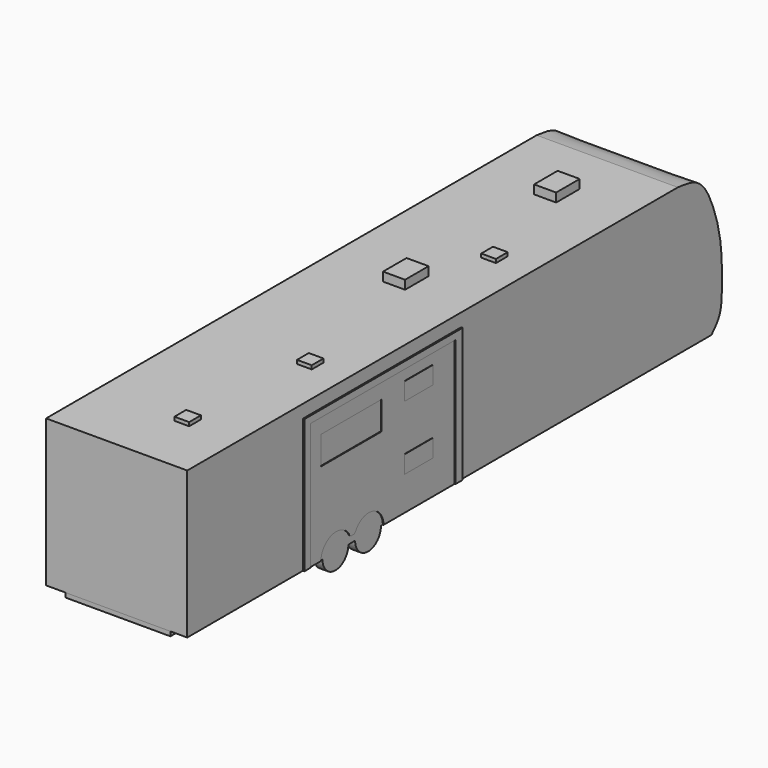
from build123d import *

# Parameters (mm, degrees)
F0_W          = 11582.4
F0_H          = 2540
F1_DEPTH      = 2438.4
F3_DEPTH      = 2438.401
F4_W          = 1738.7323379517
F4_H          = 1235.3963851929
F4_W_2        = 1517.0154571533
F4_H_2        = 1050.2412319183
F5_DEPTH      = 25.4
F4_W_3        = 98.7977981567
F4_H_3        = 270.7209965363
F4_W_4        = 115.3562068939
F4_W_5        = 121.3853359222
F4_W_6        = 111.6482615471
F6_DEPTH      = 25.4
F4_W_7        = 1592.5345420837
F4_H_4        = 643.6148881912
F4_W_8        = 1699.8038291931
F4_W_9        = 1669.4720983505
F4_H_5        = 1913.9534341023
F4_W_10       = 1458.6684703827
F4_H_6        = 455.104470253
F4_W_11       = 1482.0072054863
F4_H_7        = 385.0883245468
F7_DEPTH      = 12.7
F8_R          = 5.08
F9_DEPTH      = 152.4
F11_DEPTH     = 25.4
F10_W         = 1309.9219799042
F10_H         = 488.621711731
F12_DEPTH     = 12.7
F13_DEPTH     = 152.4
F16_W         = 609.6
F16_H         = 304.8
F17_DEPTH     = 6.35
F18_W         = 381
F18_H         = 508
F19_DEPTH     = 152.4
F20_W         = 381
F20_H         = 508
F21_DEPTH     = 152.4
F22_W         = 254
F22_H         = 254
F23_DEPTH     = 63.5
F24_DEPTH     = 76.2
F25_W         = 1815.4902458191
F25_H         = 11320.1663866639
F26_DEPTH     = 76.2
F27_W         = 1015.8215761185
F27_H         = 287.8160476685
F28_DEPTH     = 812.8
F29_R         = 48.2426226407
F29_W         = 291.1487817764
F29_H         = 228.4393310547
F30_DEPTH     = 2692.401
F31_DEPTH     = 1016
F32_DEPTH     = 203.2
F33_W         = 109.7394227982
F33_H         = 105.7481765747
F34_DEPTH     = 101.6
F35_R         = 5.08
F36_T1_DEPTH  = 807.72
F36_T3_DEPTH  = 277.6560476685
F36_T5_DEPTH  = 1005.6615761185
F36_T7_DEPTH  = 280.9887817764
F36_T9_DEPTH  = 218.2793310547
F36_T11_DEPTH = 198.12
F36_S15_W     = 5.1816
F36_S15_H     = 5.1816
F36_T16_DEPTH = 5.1816
F36_S21_W     = 5.1816
F36_S21_H     = 5.1816
F36_T22_DEPTH = 5.1816
F36_S27_W     = 5.1816
F36_S27_H     = 5.1816
F36_T28_DEPTH = 5.1816
F36_S33_W     = 5.1816
F36_S33_H     = 5.1816
F36_T34_DEPTH = 5.1816
F36_S39_W     = 5.1816
F36_S39_H     = 5.1816
F36_T40_DEPTH = 5.1816
F36_S45_W     = 5.1816
F36_S45_H     = 5.1816
F36_T46_DEPTH = 5.1816
F36_S51_W     = 5.1816
F36_S51_H     = 5.1816
F36_T52_DEPTH = 5.1816
F36_S57_W     = 5.1816
F36_S57_H     = 5.1816
F36_T58_DEPTH = 5.1816


# Not quite as in the source:
# - a fillet or chamfer that OpenCascade refuses, or shapes differently, is made with other operations: its cross-section is extruded or revolved along the edge and cut away or added


with BuildPart() as f1:
    # F0 (on Right) → F1 (new body)
    with BuildSketch(Plane.YZ):
        with Locations((5698.256055963, 1234.2060510814)):
            Rectangle(F0_W, F0_H)
    extrude(amount=F1_DEPTH)

    # F2 (on face) → F3 (cut, through all)
    with BuildSketch(Plane.YZ.offset(2438.4)):
        with BuildLine():
            add(Edge.make_bspline(
                [(11227.222442627, -35.7939489186), (11294.0039001697, 34.5419059531), (11441.1259256499, 189.4944004532), (11456.5368861302, 627.4797591897), (11449.8051343447, 1303.5662571069), (11282.6522390087, 1895.0626876843), (11004.4375304796, 2451.3086370719), (10662.2814417447, 2487.1113814171), (10498.9128112793, 2504.2060510814)],
                knots=[0, 0, 0, 0, 0.1266930612, 0.2791095084, 0.4735188477, 0.6617102021, 0.8384774002, 1, 1, 1, 1], degree=3))
            Line((11227.222442627, -35.7939489186), (11489.456055963, -35.7939489186))
            Line((11489.456055963, -35.7939489186), (11489.456055963, 2504.2060510814))
            Line((11489.456055963, 2504.2060510814), (10498.9128112793, 2504.2060510814))
        make_face()
    extrude(amount=-F3_DEPTH, mode=Mode.SUBTRACT)

    # F4 (on face) → F5 (join)
    with BuildSketch(Plane(origin=(0, 0, 0), x_dir=(0, -1, 0), z_dir=(-1, 0, 0))):
        with Locations((-9058.8221549988, 1646.3215351105)):
            Rectangle(F4_W, F4_H)
        with Locations((-9064.6572113037, 1647.0986604691)):
            Rectangle(F4_W_2, F4_H_2, mode=Mode.SUBTRACT)
        Polygon((-6864.5935058594, 234.9270476177), (-6765.7957077026, 234.9270476177), (-6765.7957077026, 2148.88048172), (-5554.6798706055, 2148.88048172), (-2582.3545455933, 2148.88048172), (-2582.3545455933, 234.9270476177), (-2466.9983386993, 234.9270476177), (-2466.9983386993, 2264.0197277069), (-6864.5935058594, 2264.0197277069), align=None)
        Polygon((-2196.6965198517, 2264.0197277069), (-2196.6965198517, 234.9270476177), (-2075.3111839294, 234.9270476177), (-2075.3111839294, 2148.88048172), (-405.8390855789, 2148.88048172), (-405.8390855789, 234.9270476177), (-294.1908240318, 234.9270476177), (-294.1908240318, 2264.0197277069), align=None)
    extrude(amount=F5_DEPTH)

    # F4 (on face) + F5_face (on face) → F6 (join)
    with BuildSketch(Plane(origin=(0, 0, 0), x_dir=(0, -1, 0), z_dir=(-1, 0, 0))):
        with Locations((-6815.194606781, 99.5665493496)):
            Rectangle(F4_W_3, F4_H_3)
        with Locations((-2524.6764421463, 99.5665493496)):
            Rectangle(F4_W_4, F4_H_3)
        with Locations((-2136.0038518906, 99.5665493496)):
            Rectangle(F4_W_5, F4_H_3)
        with Locations((-350.0149548054, 99.5665493496)):
            Rectangle(F4_W_6, F4_H_3)
    with BuildSketch(Plane(origin=(-25.4, 4593.443098287, 1752.5802822759), x_dir=(0, -1, 0), z_dir=(-1, 0, 0))):
        Polygon((-2271.1504075724, -1517.6532346582), (-2172.3526094156, -1517.6532346582), (-2172.3526094156, 396.3001994441), (2011.0885526937, 396.3001994441), (2011.0885526937, -1517.6532346582), (2126.4447595877, -1517.6532346582), (2126.4447595877, 511.439445431), (-2271.1504075724, 511.439445431), align=None)
        Polygon((2396.7465784353, 511.439445431), (2396.7465784353, -1517.6532346582), (2518.1319143576, -1517.6532346582), (2518.1319143576, 396.3001994441), (4187.6040127081, 396.3001994441), (4187.6040127081, -1517.6532346582), (4299.2522742552, -1517.6532346582), (4299.2522742552, 511.439445431), align=None)
    extrude(amount=F6_DEPTH)

    # F4 (on face) → F7 (join)
    with BuildSketch(Plane(origin=(0, 0, 0), x_dir=(0, -1, 0), z_dir=(-1, 0, 0))):
        with BuildLine():
            Line((-6765.7957077026, 2148.88048172), (-6765.7957077026, 234.9270476177))
            Line((-6765.7957077026, 234.9270476177), (-3972.2290414832, 234.9270476177))
            ThreePointArc((-3972.2290414832, 234.9270476177), (-3810.8091471396, 279.2122748766), (-3649.3892527959, 234.9270476177))
            Line((-3649.3892527959, 234.9270476177), (-3268.7322256311, 234.9270476177))
            ThreePointArc((-3268.7322256311, 234.9270476177), (-3106.7426501641, 278.4144938222), (-2944.7530746971, 234.9270476177))
            Line((-2944.7530746971, 234.9270476177), (-2582.3545455933, 234.9270476177))
            Line((-2582.3545455933, 234.9270476177), (-2582.3545455933, 2148.88048172))
            Line((-2582.3545455933, 2148.88048172), (-5554.6798706055, 2148.88048172))
            Line((-5554.6798706055, 2148.88048172), (-6765.7957077026, 2148.88048172))
        make_face()
        with Locations((-5719.4011211395, 1632.1941018105)):
            Rectangle(F4_W_7, F4_H_4, mode=Mode.SUBTRACT)
        with Locations((-3710.1671695709, 1632.1941018105)):
            Rectangle(F4_W_8, F4_H_4, mode=Mode.SUBTRACT)
        with BuildLine():
            Line((-3972.2290414832, 234.9270476177), (-6765.7957077026, 234.9270476177))
            Line((-6765.7957077026, 234.9270476177), (-6765.7957077026, -35.7939489186))
            Line((-6765.7957077026, -35.7939489186), (-4127.1371841431, -35.7939489186))
            ThreePointArc((-4127.1371841431, -35.7939489186), (-4085.3692242957, 119.9863517264), (-3972.2290414832, 234.9270476177))
        make_face()
        with BuildLine():
            Line((-2582.3545455933, 234.9270476177), (-2944.7530746971, 234.9270476177))
            ThreePointArc((-2944.7530746971, 234.9270476177), (-2828.889020926, 120.5433614824), (-2783.4274768829, -35.7939489186))
            Line((-2783.4274768829, -35.7939489186), (-2582.3545455933, -35.7939489186))
            Line((-2582.3545455933, -35.7939489186), (-2582.3545455933, 234.9270476177))
        make_face()
        with Locations((-1240.5751347542, 99.5665493496)):
            Rectangle(F4_W_9, F4_H_3)
        with Locations((-1240.5751347542, 1191.9037646688)):
            Rectangle(F4_W_9, F4_H_5)
        with Locations((-1246.5664148331, 1260.11043787)):
            Rectangle(F4_W_10, F4_H_6, mode=Mode.SUBTRACT)
        with Locations((-1246.5664446354, 1855.2470803261)):
            Rectangle(F4_W_11, F4_H_7, mode=Mode.SUBTRACT)
        with Locations((-9064.6572113037, 1647.0986604691)):
            Rectangle(F4_W_2, F4_H_2)
    extrude(amount=F7_DEPTH)

    # F8
    f8_edges = [f1.edges().sort_by_distance(p)[0] for p in [
        (-12.7, 1987.570047, 1855.24708),
        (-12.7, 1246.566445, 2047.791243),
    ]]
    fillet(f8_edges, radius=F8_R)

    # F4 (on face) → F9 (join)
    with BuildSketch(Plane(origin=(0, 0, 0), x_dir=(0, -1, 0), z_dir=(-1, 0, 0))):
        with BuildLine():
            ThreePointArc((-3528.5879283905, -35.7939489186), (-3807.9879283905, 243.6060510814), (-4087.3879283905, -35.7939489186))
            Line((-4087.3879283905, -35.7939489186), (-3528.5879283905, -35.7939489186))
        make_face()
        with BuildLine():
            Line((-3528.5879283905, -35.7939489186), (-4087.3879283905, -35.7939489186))
            ThreePointArc((-4087.3879283905, -35.7939489186), (-3807.9879283905, -315.1939489186), (-3528.5879283905, -35.7939489186))
        make_face()
        with BuildLine():
            Line((-2828.4271865845, -35.7939489186), (-3387.2271865845, -35.7939489186))
            ThreePointArc((-3387.2271865845, -35.7939489186), (-3107.8271865845, -315.1939489186), (-2828.4271865845, -35.7939489186))
        make_face()
        with BuildLine():
            ThreePointArc((-2828.4271865845, -35.7939489186), (-3107.8271865845, 243.6060510814), (-3387.2271865845, -35.7939489186))
            Line((-3387.2271865845, -35.7939489186), (-2828.4271865845, -35.7939489186))
        make_face()
    extrude(amount=-F9_DEPTH)

    # F10 (on face) → F11 (join)
    with BuildSketch(Plane.YZ.offset(2438.4)):
        Polygon((5663.0005836487, 83.0691084266), (5663.4521484375, -35.7939489186), (5820.454120636, -35.7939489186), (5820.454120636, 231.9672825278), (5663.0005836487, 231.9672825278), align=None)
        Polygon((2402.78840065, -35.7939489186), (2534.1942310333, -35.7939489186), (2541.718006134, 83.0691084266), (2541.718006134, 231.9672825278), (2402.78840065, 231.9672825278), align=None)
        Polygon((2402.78840065, 231.9672825278), (2541.718006134, 231.9672825278), (2541.718006134, 2157.7496528625), (5663.0005836487, 2157.7496528625), (5663.0005836487, 231.9672825278), (5820.454120636, 231.9672825278), (5820.454120636, 2278.1553268433), (2402.78840065, 2278.1553268433), align=None)
    extrude(amount=F11_DEPTH)

    # F10 (on face) → F12 (join)
    with BuildSketch(Plane.YZ.offset(2438.4)):
        with BuildLine():
            Line((2541.718006134, 231.9672825278), (2935.8405070918, 231.9672825278))
            ThreePointArc((2935.8405070918, 231.9672825278), (3105.7881003582, 278.912424909), (3275.7356936245, 231.9672825278))
            Line((3275.7356936245, 231.9672825278), (3637.7238895078, 231.9672825278))
            ThreePointArc((3637.7238895078, 231.9672825278), (3807.7616169979, 280.4213909384), (3977.799344488, 231.9672825278))
            Line((3977.7993444881, 231.9672825278), (5663.0005836487, 231.9672825278))
            Line((5663.0005836487, 231.9672825278), (5663.0005836487, 2157.7496528625))
            Line((5663.0005836487, 2157.7496528625), (2541.718006134, 2157.7496528625))
            Line((2541.718006134, 2157.7496528625), (2541.718006134, 231.9672825278))
        make_face()
        with Locations((3433.8718652725, 1646.3187932968)):
            Rectangle(F10_W, F10_H, mode=Mode.SUBTRACT)
        with BuildLine():
            Line((2534.1942310333, -35.7939489186), (2775.1047611237, -35.7939489186))
            ThreePointArc((2775.1047611237, -35.7939489186), (2821.9186727852, 118.2289442144), (2935.8405070918, 231.9672825278))
            Line((2935.8405070918, 231.9672825278), (2541.718006134, 231.9672825278))
            Line((2541.718006134, 231.9672825278), (2541.718006134, 83.0691084266))
            Line((2541.718006134, 83.0691084266), (2534.1942310333, -35.7939489186))
        make_face()
        with BuildLine():
            Line((3637.7238895078, 231.9672825278), (3275.7356936245, 231.9672825278))
            ThreePointArc((3275.7356936245, 231.9672825278), (3332.4353980139, 189.1756777604), (3378.7021636963, 135.274246335))
            ThreePointArc((3378.7021636963, 135.274246335), (3398.1239015568, 103.4115989251), (3429.4067288236, 83.0691084266))
            Line((3429.4067288236, 83.0691084266), (3487.6588915988, 83.0691084266))
            ThreePointArc((3487.6588915988, 83.0691084266), (3518.9417188656, 103.4115989251), (3538.3634567261, 135.274246335))
            ThreePointArc((3538.3634567261, 135.274246335), (3582.7874836507, 189.021952363), (3637.7238895078, 231.9672825278))
        make_face()
        with BuildLine():
            ThreePointArc((3977.799344488, 231.9672825278), (4088.076710876, 117.4697924054), (4130.2785873413, -35.7939489186))
            Line((4130.2785873413, -35.7939489186), (5663.4521484375, -35.7939489186))
            Line((5663.4521484375, -35.7939489186), (5663.0005836487, 83.0691084266))
            Line((5663.0005836487, 83.0691084266), (5663.0005836487, 231.9672825278))
            Line((5663.0005836487, 231.9672825278), (3977.7993444881, 231.9672825278))
        make_face()
    extrude(amount=F12_DEPTH)

    # F10 (on face) → F13 (join)
    with BuildSketch(Plane.YZ.offset(2438.4)):
        with BuildLine():
            ThreePointArc((2826.7098575592, -35.7939489186), (3106.1098575592, -315.1939489186), (3385.5098575592, -35.7939489186))
            Line((3385.5098575592, -35.7939489186), (2826.7098575592, -35.7939489186))
        make_face()
        with BuildLine():
            Line((2826.7098575592, -35.7939489186), (3385.5098575592, -35.7939489186))
            ThreePointArc((3385.5098575592, -35.7939489186), (3106.1098575592, 243.6060510814), (2826.7098575592, -35.7939489186))
        make_face()
        with BuildLine():
            ThreePointArc((4090.3557628632, -35.7939489186), (3810.9557628632, 243.6060510814), (3531.5557628632, -35.7939489186))
            Line((3531.5557628632, -35.7939489186), (4090.3557628632, -35.7939489186))
        make_face()
        with BuildLine():
            Line((4090.3557628632, -35.7939489186), (3531.5557628632, -35.7939489186))
            ThreePointArc((3531.5557628632, -35.7939489186), (3810.9557628632, -315.1939489186), (4090.3557628632, -35.7939489186))
        make_face()
    extrude(amount=-F13_DEPTH)

    # F16 (on face) → F17 (join)
    with BuildSketch(Plane.YZ.offset(2451.1)):
        with Locations((4881.9495035825, 1817.1032423055)):
            Rectangle(F16_W, F16_H)
        with Locations((4881.9495035825, 706.4627090574)):
            Rectangle(F16_W, F16_H)
    extrude(amount=F17_DEPTH)

    # F18 (on face) → F19 (join)
    with BuildSketch(Plane.XY.offset(2504.2060510814)):
        with Locations((1243.6975836754, 9382.0020343422)):
            Rectangle(F18_W, F18_H)
    extrude(amount=F19_DEPTH)

    # F20 (on face) → F21 (join)
    with BuildSketch(Plane.XY.offset(2504.2060510814)):
        with Locations((1243.6975836754, 6119.3277945057)):
            Rectangle(F20_W, F20_H)
    extrude(amount=F21_DEPTH)

    # F22 (on face) → F23 (join)
    with BuildSketch(Plane.XY.offset(2504.2060510814)):
        with Locations((1778.1576690674, 7366.1090393066)):
            Rectangle(F22_W, F22_H)
        with Locations((1778.1576690674, 3388.5683078766)):
            Rectangle(F22_W, F22_H)
        with Locations((1524.1576690674, 1059.3781728745)):
            Rectangle(F22_W, F22_H)
    extrude(amount=F23_DEPTH)

    # F29 (on face) → F30 (cut, through all)
    with BuildSketch(Plane(origin=(0, 0, -35.7939489186), x_dir=(1, 0, 0), z_dir=(0, 0, -1))):
        with Locations((1222.6868448267, -12362.519959551)):
            Circle(F29_R)
        with Locations((1216.6296839714, -12109.4274520874)):
            Rectangle(F29_W, F29_H)
    extrude(amount=-F30_DEPTH, mode=Mode.SUBTRACT)


with BuildPart() as f24:
    # F14 (on face) → F24 (new body)
    with BuildSketch(Plane(origin=(0, 0, -35.7939489186), x_dir=(1, 0, 0), z_dir=(0, 0, -1))):
        Polygon((1219.2, -11227.222442627), (304.5125207247, -11227.222442627), (1230.4298877716, -12745.1028823853), (2156.3472548186, -11227.222442627), align=None)
    extrude(amount=F24_DEPTH)

    # F27 (on face) → F28 (join)
    with BuildSketch(Plane(origin=(0, 0, -35.7939489186), x_dir=(1, 0, 0), z_dir=(0, 0, -1))):
        with Locations((1225.6785035133, -11765.1133537292)):
            Rectangle(F27_W, F27_H)
    extrude(amount=-F28_DEPTH)

    # F29 (on face) → F31 (join)
    with BuildSketch(Plane(origin=(0, 0, -35.7939489186), x_dir=(1, 0, 0), z_dir=(0, 0, -1))):
        with BuildLine():
            ThreePointArc((1230.3896392389, -12314.8962511959), (1185.9516189301, -12393.7909335936), (1270.9294674674, -12362.519959551))
            ThreePointArc((1270.9294674674, -12362.519959551), (1259.4220707233, -12331.2489855084), (1230.3896392389, -12314.8962511959))
        make_face()
    extrude(amount=-F31_DEPTH)

    # F29 (on face) → F32 (join)
    with BuildSketch(Plane(origin=(0, 0, -35.7939489186), x_dir=(1, 0, 0), z_dir=(0, 0, -1))):
        with Locations((1222.6868448267, -12362.519959551)):
            Circle(F29_R)
        with Locations((1216.6296839714, -12109.4274520874)):
            Rectangle(F29_W, F29_H)
    extrude(amount=-F32_DEPTH)

    # F33 (on face) → F34 (join)
    with BuildSketch(Plane.XY.offset(980.2060510814)):
        with Locations((1221.1564183235, 12363.9168739319)):
            Rectangle(F33_W, F33_H)
    extrude(amount=F34_DEPTH)

    # F35
    f35_edges = [f24.edges().sort_by_distance(p)[0] for p in [
        (1276.02613, 12416.790962, 1031.006051),
        (1276.02613, 12311.042786, 1031.006051),
        (1276.02613, 12363.916874, 1081.806051),
        (1221.156418, 12416.790962, 1081.806051),
        (1166.286707, 12363.916874, 1081.806051),
        (1221.156418, 12311.042786, 1081.806051),
        (1166.286707, 12311.042786, 1031.006051),
        (1166.286707, 12416.790962, 1031.006051),
    ]]
    fillet(f35_edges, radius=F35_R)

    # F36: fillet of radius 5.08 on 16 edges, made by hand

    # F36_s2 → F36_t1 (cut)
    with BuildSketch(Plane.XY.offset(-35.7939489186)):
        with BuildLine():
            ThreePointArc((717.7677154541, 11903.9413775635), (719.2556130057, 11907.5334800119), (722.8477154541, 11909.0213775635))
            Line((722.8477154541, 11909.0213775635), (717.7677154541, 11909.0213775635))
            Line((717.7677154541, 11909.0213775635), (717.7677154541, 11903.9413775635))
        make_face()
        with BuildLine():
            ThreePointArc((717.7677154541, 11626.285329895), (719.2556130057, 11622.6932274466), (722.8477154541, 11621.205329895))
            Line((722.8477154541, 11621.205329895), (717.7677154541, 11621.205329895))
            Line((717.7677154541, 11621.205329895), (717.7677154541, 11626.285329895))
        make_face()
        with BuildLine():
            ThreePointArc((1728.5092915726, 11909.0213775635), (1732.101394021, 11907.5334800119), (1733.5892915726, 11903.9413775635))
            Line((1733.5892915726, 11903.9413775635), (1733.5892915726, 11909.0213775635))
            Line((1733.5892915726, 11909.0213775635), (1728.5092915726, 11909.0213775635))
        make_face()
        with BuildLine():
            ThreePointArc((1728.5092915726, 11621.205329895), (1732.101394021, 11622.6932274466), (1733.5892915726, 11626.285329895))
            Line((1733.5892915726, 11626.285329895), (1733.5892915726, 11621.205329895))
            Line((1733.5892915726, 11621.205329895), (1728.5092915726, 11621.205329895))
        make_face()
    extrude(amount=F36_T1_DEPTH, mode=Mode.SUBTRACT)

    # F36_s4 → F36_t3 (cut)
    with BuildSketch(Plane.XZ.offset(-11903.9413775635)):
        with BuildLine():
            ThreePointArc((717.7677154541, 771.9260510814), (719.2556130057, 775.5181535298), (722.8477154541, 777.0060510814))
            Line((722.8477154541, 777.0060510814), (717.7677154541, 777.0060510814))
            Line((717.7677154541, 777.0060510814), (717.7677154541, 771.9260510814))
        make_face()
        with BuildLine():
            ThreePointArc((1733.5892915726, 771.9260510814), (1732.101394021, 775.5181535298), (1728.5092915726, 777.0060510814))
            Line((1728.5092915726, 777.0060510814), (1733.5892915726, 777.0060510814))
            Line((1733.5892915726, 777.0060510814), (1733.5892915726, 771.9260510814))
        make_face()
    extrude(amount=F36_T3_DEPTH, mode=Mode.SUBTRACT)

    # F36_s6 → F36_t5 (cut)
    with BuildSketch(Plane.YZ.offset(722.8477154541)):
        with BuildLine():
            ThreePointArc((11621.205329895, 771.9260510814), (11622.6932274466, 775.5181535298), (11626.285329895, 777.0060510814))
            Line((11626.285329895, 777.0060510814), (11621.205329895, 777.0060510814))
            Line((11621.205329895, 777.0060510814), (11621.205329895, 771.9260510814))
        make_face()
        with BuildLine():
            ThreePointArc((11909.0213775635, 771.9260510814), (11907.5334800119, 775.5181535298), (11903.9413775635, 777.0060510814))
            Line((11903.9413775635, 777.0060510814), (11909.0213775635, 777.0060510814))
            Line((11909.0213775635, 777.0060510814), (11909.0213775635, 771.9260510814))
        make_face()
    extrude(amount=F36_T5_DEPTH, mode=Mode.SUBTRACT)

    # F36_s8 → F36_t7 (cut)
    with BuildSketch(Plane.YZ.offset(1076.1352930832)):
        with BuildLine():
            ThreePointArc((11995.2077865601, 162.3260510814), (11996.6956841116, 165.9181535298), (12000.2877865601, 167.4060510814))
            Line((12000.2877865601, 167.4060510814), (11995.2077865601, 167.4060510814))
            Line((11995.2077865601, 167.4060510814), (11995.2077865601, 162.3260510814))
        make_face()
        with BuildLine():
            ThreePointArc((12223.6471176147, 162.3260510814), (12222.1592200632, 165.9181535298), (12218.5671176147, 167.4060510814))
            Line((12218.5671176147, 167.4060510814), (12223.6471176147, 167.4060510814))
            Line((12223.6471176147, 167.4060510814), (12223.6471176147, 162.3260510814))
        make_face()
    extrude(amount=F36_T7_DEPTH, mode=Mode.SUBTRACT)

    # F36_s10 → F36_t9 (cut)
    with BuildSketch(Plane.XZ.offset(-12218.5671176147)):
        with BuildLine():
            ThreePointArc((1071.0552930832, 162.3260510814), (1072.5431906348, 165.9181535298), (1076.1352930832, 167.4060510814))
            Line((1076.1352930832, 167.4060510814), (1071.0552930832, 167.4060510814))
            Line((1071.0552930832, 167.4060510814), (1071.0552930832, 162.3260510814))
        make_face()
        with BuildLine():
            ThreePointArc((1362.2040748596, 162.3260510814), (1360.716177308, 165.9181535298), (1357.1240748596, 167.4060510814))
            Line((1357.1240748596, 167.4060510814), (1362.2040748596, 167.4060510814))
            Line((1362.2040748596, 167.4060510814), (1362.2040748596, 162.3260510814))
        make_face()
    extrude(amount=F36_T9_DEPTH, mode=Mode.SUBTRACT)

    # F36_s12 → F36_t11 (cut)
    with BuildSketch(Plane.XY.offset(-35.7939489186)):
        with BuildLine():
            ThreePointArc((1071.0552930832, 12000.2877865601), (1072.5431906348, 11996.6956841116), (1076.1352930832, 11995.2077865601))
            Line((1076.1352930832, 11995.2077865601), (1071.0552930832, 11995.2077865601))
            Line((1071.0552930832, 11995.2077865601), (1071.0552930832, 12000.2877865601))
        make_face()
        with BuildLine():
            ThreePointArc((1071.0552930832, 12218.5671176147), (1072.5431906348, 12222.1592200632), (1076.1352930832, 12223.6471176147))
            Line((1076.1352930832, 12223.6471176147), (1071.0552930832, 12223.6471176147))
            Line((1071.0552930832, 12223.6471176147), (1071.0552930832, 12218.5671176147))
        make_face()
        with BuildLine():
            ThreePointArc((1357.1240748596, 12223.6471176147), (1360.716177308, 12222.1592200632), (1362.2040748596, 12218.5671176147))
            Line((1362.2040748596, 12218.5671176147), (1362.2040748596, 12223.6471176147))
            Line((1362.2040748596, 12223.6471176147), (1357.1240748596, 12223.6471176147))
        make_face()
        with BuildLine():
            ThreePointArc((1362.2040748596, 12000.2877865601), (1360.716177308, 11996.6956841116), (1357.1240748596, 11995.2077865601))
            Line((1357.1240748596, 11995.2077865601), (1362.2040748596, 11995.2077865601))
            Line((1362.2040748596, 11995.2077865601), (1362.2040748596, 12000.2877865601))
        make_face()
    extrude(amount=F36_T11_DEPTH, mode=Mode.SUBTRACT)


with BuildPart() as f26:
    # F25 (on face) → F26 (new body)
    with BuildSketch(Plane(origin=(0, 0, -35.7939489186), x_dir=(1, 0, 0), z_dir=(0, 0, -1))):
        with Locations((1239.3982410431, -5567.139249295)):
            Rectangle(F25_W, F25_H)
    extrude(amount=F26_DEPTH)


with BuildPart() as f36_tool14:
    # F36_s15 → F36_t16 (new body)
    with BuildSketch(Plane.XZ.offset(-11903.9413775635)):
        with Locations((720.2569154541, 774.5168510814)):
            Rectangle(F36_S15_W, F36_S15_H)
    extrude(amount=-F36_T16_DEPTH)

    # F36_s17 → F36_t18 (revolve, cut)
    with BuildSketch(Plane(origin=(722.8477154541, 11903.9413775635, 771.9260510814), x_dir=(0.7071067812, 0, -0.7071067812), z_dir=(0.7071067812, 0, 0.7071067812))):
        with BuildLine():
            ThreePointArc((0, -5.08), (5.08, 0), (0, 5.08))
            Line((0, 5.08), (0, -5.08))
        make_face()
    revolve(axis=Axis((722.8477154541, 11903.9413775635, 771.9260510814), (0, 1, 0)), mode=Mode.SUBTRACT)


with BuildPart() as f24_1:
    add(f24.part)

    # F36_t13: cut F36_tool14
    add(f36_tool14.part, mode=Mode.SUBTRACT)


with BuildPart() as f36_tool20:
    # F36_s21 → F36_t22 (new body)
    with BuildSketch(Plane.XY.offset(771.9260510814)):
        with Locations((720.2569154541, 11623.694529895)):
            Rectangle(F36_S21_W, F36_S21_H)
    extrude(amount=F36_T22_DEPTH)

    # F36_s23 → F36_t24 (revolve, cut)
    with BuildSketch(Plane(origin=(722.8477154541, 11626.285329895, 771.9260510814), x_dir=(0.7071067812, 0.7071067812, 0), z_dir=(0.7071067812, -0.7071067812, 0))):
        with BuildLine():
            ThreePointArc((0, -5.08), (5.08, 0), (0, 5.08))
            Line((0, 5.08), (0, -5.08))
        make_face()
    revolve(axis=Axis((722.8477154541, 11626.285329895, 771.9260510814), (0, 0, 1)), mode=Mode.SUBTRACT)


with BuildPart() as f24_2:
    add(f24_1.part)

    # F36_t19: cut F36_tool20
    add(f36_tool20.part, mode=Mode.SUBTRACT)


with BuildPart() as f36_tool26:
    # F36_s27 → F36_t28 (new body)
    with BuildSketch(Plane.XZ.offset(-11626.285329895)):
        with Locations((1731.1000915726, 774.5168510814)):
            Rectangle(F36_S27_W, F36_S27_H)
    extrude(amount=F36_T28_DEPTH)

    # F36_s29 → F36_t30 (revolve, cut)
    with BuildSketch(Plane(origin=(1728.5092915726, 11626.285329895, 771.9260510814), x_dir=(-0.7071067812, 0, -0.7071067812), z_dir=(-0.7071067812, 0, 0.7071067812))):
        with BuildLine():
            ThreePointArc((0, -5.08), (5.08, 0), (0, 5.08))
            Line((0, 5.08), (0, -5.08))
        make_face()
    revolve(axis=Axis((1728.5092915726, 11626.285329895, 771.9260510814), (0, -1, 0)), mode=Mode.SUBTRACT)


with BuildPart() as f24_3:
    add(f24_2.part)

    # F36_t25: cut F36_tool26
    add(f36_tool26.part, mode=Mode.SUBTRACT)


with BuildPart() as f36_tool32:
    # F36_s33 → F36_t34 (new body)
    with BuildSketch(Plane.XZ.offset(-11903.9413775635)):
        with Locations((1731.1000915726, 774.5168510814)):
            Rectangle(F36_S33_W, F36_S33_H)
    extrude(amount=-F36_T34_DEPTH)

    # F36_s35 → F36_t36 (revolve, cut)
    with BuildSketch(Plane(origin=(1728.5092915726, 11903.9413775635, 771.9260510814), x_dir=(-0.7071067812, 0, -0.7071067812), z_dir=(0.7071067812, 0, -0.7071067812))):
        with BuildLine():
            ThreePointArc((0, -5.08), (5.08, 0), (0, 5.08))
            Line((0, 5.08), (0, -5.08))
        make_face()
    revolve(axis=Axis((1728.5092915726, 11903.9413775635, 771.9260510814), (0, 1, 0)), mode=Mode.SUBTRACT)


with BuildPart() as f24_4:
    add(f24_3.part)

    # F36_t31: cut F36_tool32
    add(f36_tool32.part, mode=Mode.SUBTRACT)


with BuildPart() as f36_tool38:
    # F36_s39 → F36_t40 (new body)
    with BuildSketch(Plane.XY.offset(162.3260510814)):
        with Locations((1359.7148748596, 11997.6969865601)):
            Rectangle(F36_S39_W, F36_S39_H)
    extrude(amount=F36_T40_DEPTH)

    # F36_s41 → F36_t42 (revolve, cut)
    with BuildSketch(Plane(origin=(1357.1240748596, 12000.2877865601, 162.3260510814), x_dir=(-0.7071067812, 0.7071067812, 0), z_dir=(0.7071067812, 0.7071067812, 0))):
        with BuildLine():
            ThreePointArc((0, -5.08), (5.08, 0), (0, 5.08))
            Line((0, 5.08), (0, -5.08))
        make_face()
    revolve(axis=Axis((1357.1240748596, 12000.2877865601, 162.3260510814), (0, 0, 1)), mode=Mode.SUBTRACT)


with BuildPart() as f24_5:
    add(f24_4.part)

    # F36_t37: cut F36_tool38
    add(f36_tool38.part, mode=Mode.SUBTRACT)


with BuildPart() as f36_tool44:
    # F36_s45 → F36_t46 (new body)
    with BuildSketch(Plane.XY.offset(162.3260510814)):
        with Locations((1073.5444930832, 11997.6969865601)):
            Rectangle(F36_S45_W, F36_S45_H)
    extrude(amount=F36_T46_DEPTH)

    # F36_s47 → F36_t48 (revolve, cut)
    with BuildSketch(Plane(origin=(1076.1352930832, 12000.2877865601, 162.3260510814), x_dir=(0.7071067812, 0.7071067812, 0), z_dir=(0.7071067812, -0.7071067812, 0))):
        with BuildLine():
            ThreePointArc((0, -5.08), (5.08, 0), (0, 5.08))
            Line((0, 5.08), (0, -5.08))
        make_face()
    revolve(axis=Axis((1076.1352930832, 12000.2877865601, 162.3260510814), (0, 0, 1)), mode=Mode.SUBTRACT)


with BuildPart() as f24_6:
    add(f24_5.part)

    # F36_t43: cut F36_tool44
    add(f36_tool44.part, mode=Mode.SUBTRACT)


with BuildPart() as f36_tool50:
    # F36_s51 → F36_t52 (new body)
    with BuildSketch(Plane.XY.offset(162.3260510814)):
        with Locations((1073.5444930832, 12221.1579176147)):
            Rectangle(F36_S51_W, F36_S51_H)
    extrude(amount=F36_T52_DEPTH)

    # F36_s53 → F36_t54 (revolve, cut)
    with BuildSketch(Plane(origin=(1076.1352930832, 12218.5671176147, 162.3260510814), x_dir=(0.7071067812, -0.7071067812, 0), z_dir=(-0.7071067812, -0.7071067812, 0))):
        with BuildLine():
            ThreePointArc((0, -5.08), (5.08, 0), (0, 5.08))
            Line((0, 5.08), (0, -5.08))
        make_face()
    revolve(axis=Axis((1076.1352930832, 12218.5671176147, 162.3260510814), (0, 0, 1)), mode=Mode.SUBTRACT)


with BuildPart() as f24_7:
    add(f24_6.part)

    # F36_t49: cut F36_tool50
    add(f36_tool50.part, mode=Mode.SUBTRACT)


with BuildPart() as f36_tool56:
    # F36_s57 → F36_t58 (new body)
    with BuildSketch(Plane.XY.offset(162.3260510814)):
        with Locations((1359.7148748596, 12221.1579176147)):
            Rectangle(F36_S57_W, F36_S57_H)
    extrude(amount=F36_T58_DEPTH)

    # F36_s59 → F36_t60 (revolve, cut)
    with BuildSketch(Plane(origin=(1357.1240748596, 12218.5671176147, 162.3260510814), x_dir=(-0.7071067812, -0.7071067812, 0), z_dir=(-0.7071067812, 0.7071067812, 0))):
        with BuildLine():
            ThreePointArc((0, -5.08), (5.08, 0), (0, 5.08))
            Line((0, 5.08), (0, -5.08))
        make_face()
    revolve(axis=Axis((1357.1240748596, 12218.5671176147, 162.3260510814), (0, 0, 1)), mode=Mode.SUBTRACT)


with BuildPart() as f24_8:
    add(f24_7.part)

    # F36_t55: cut F36_tool56
    add(f36_tool56.part, mode=Mode.SUBTRACT)


solid = Compound([f1.part, f26.part, f24_8.part])
